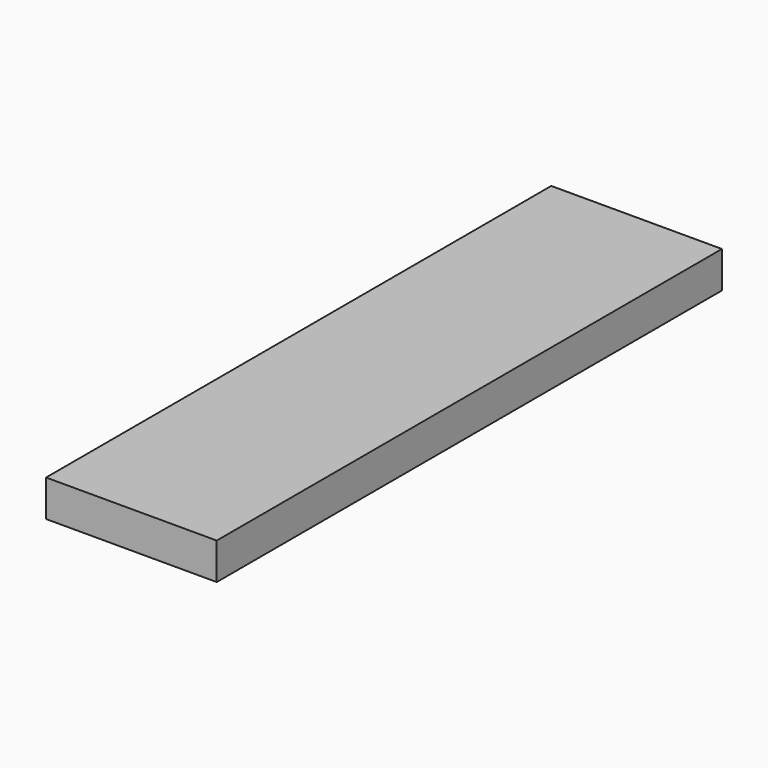
from build123d import *

# Parameters (mm, degrees)
F1_W     = 70
F1_H     = 15
F2_DEPTH = 259


with BuildPart() as f2:
    # F1 (on Front) → F2 (new body)
    with BuildSketch(Plane.XZ):
        with Locations((35, 7.5)):
            Rectangle(F1_W, F1_H)
    extrude(amount=F2_DEPTH)


solid = f2.part
